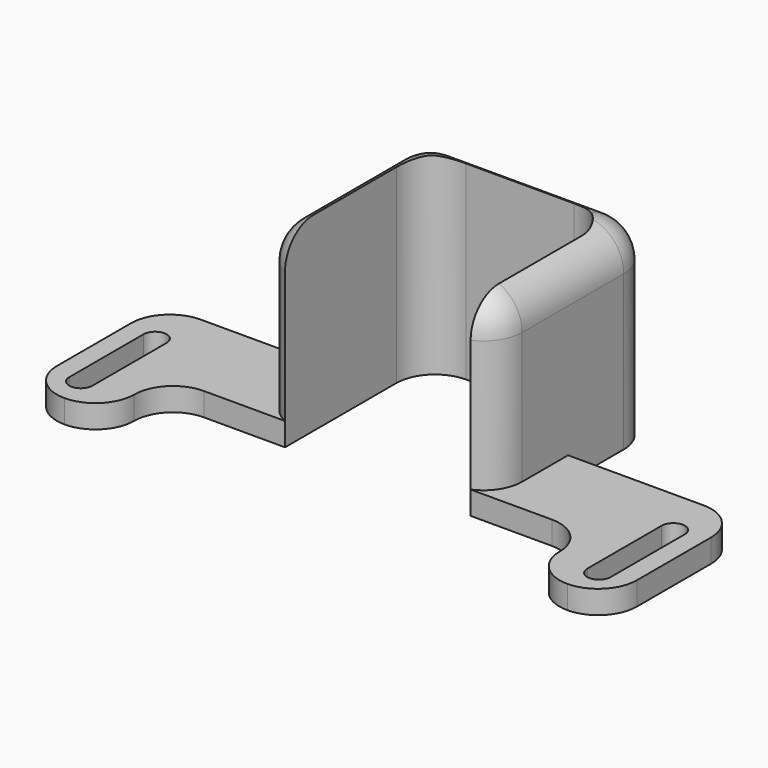
from build123d import *

# Parameters (mm, degrees)
F2_DEPTH     = 25
F3_DEPTH     = 3
F4_DEPTH     = 25
F5_R         = 4.99999
F6_T1_DEPTH  = 25
F6_T3_DEPTH  = 25
F6_T5_DEPTH  = 50
F6_T7_DEPTH  = 33.4564392374
F6_T9_DEPTH  = 50
F6_T11_DEPTH = 33.4564392374
F7_T1_DEPTH  = 16.417424305
F7_T3_DEPTH  = 20
F7_T6_ANGLE  = 89.9999999974
F7_T8_ANGLE  = 89.9999999974
F7_T10_ANGLE = 209.6926070845
F7_T12_ANGLE = 209.6926070845


# Not quite as in the source:
# - a fillet or chamfer that OpenCascade refuses, or shapes differently, is made with other operations: its cross-section is extruded or revolved along the edge and cut away or added
# - a fillet or chamfer is up to 0.001 mm smaller than in the source, because OpenCascade refuses the exact size


with BuildPart() as f2:
    # F0 (on Top) → F2 (new body)
    with BuildSketch(Plane.XY):
        Polygon((15, 36), (0, 36), (-15, 36), (-15, 22), (-15, 10), (-12, 10), (-12, 33), (0, 33), (12, 33), (12, 10), (15, 10), (15, 22), align=None)
    extrude(amount=F2_DEPTH)

    # F0 (on Top) → F3 (join)
    with BuildSketch(Plane.XY):
        Polygon((-15, 10), (-15, 22), (-37.5, 22), (-37.5, 0), (-27.5, 0), (-27.5, 10), align=None)
        Polygon((37.5, 22), (15, 22), (15, 10), (27.5, 10), (27.5, 0), (37.5, 0), align=None)
    extrude(amount=F3_DEPTH)

    # F1 (on Top) → F4 (cut)
    with BuildSketch(Plane.XY):
        with BuildLine():
            Line((35, 3.8767794613), (35, 15.8767794613))
            ThreePointArc((35, 15.8767794613), (33.5, 17.3767794613), (32, 15.8767794613))
            Line((32, 15.8767794613), (32, 3.8767794613))
            ThreePointArc((32, 3.8767794613), (33.5, 2.3767794613), (35, 3.8767794613))
        make_face()
        with BuildLine():
            ThreePointArc((-32, 15.8767794613), (-33.5, 17.3767794613), (-35, 15.8767794613))
            Line((-35, 15.8767794613), (-35, 3.8767794613))
            ThreePointArc((-35, 3.8767794613), (-33.5, 2.3767794613), (-32, 3.8767794613))
            Line((-32, 3.8767794613), (-32, 15.8767794613))
        make_face()
    extrude(amount=F4_DEPTH, mode=Mode.SUBTRACT)

    # F5 (radius 5 in the source; OpenCascade refuses exactly that, so slightly less here)
    f5_edges = [f2.edges().sort_by_distance(p)[0] for p in [
        (-37.5, 0, 1.5),
        (-27.5, 0, 1.5),
        (-37.5, 22, 1.5),
        (37.5, 22, 1.5),
        (37.5, 0, 1.5),
        (27.5, 0, 1.5),
        (27.5, 10, 1.5),
        (-27.5, 10, 1.5),
    ]]
    fillet(f5_edges, radius=F5_R)

    # F6: fillet of radius 5 on 6 edges, made by hand

    # F6_s2 → F6_t1 (join)
    with BuildSketch(Plane.XY):
        with BuildLine():
            ThreePointArc((12, 28), (10.5355339059, 31.5355339059), (7, 33))
            Line((7, 33), (12, 33))
            Line((12, 33), (12, 28))
        make_face()
    extrude(amount=F6_T1_DEPTH)

    # F6_s4 → F6_t3 (join)
    with BuildSketch(Plane.XY):
        with BuildLine():
            ThreePointArc((-7, 33), (-10.5355339059, 31.5355339059), (-12, 28))
            Line((-12, 28), (-12, 33))
            Line((-12, 33), (-7, 33))
        make_face()
    extrude(amount=F6_T3_DEPTH)

    # F6_s6 → F6_t5 (cut)
    with BuildSketch(Plane.XY.offset(-12.5)):
        with BuildLine():
            ThreePointArc((15, 31), (13.5355339059, 34.5355339059), (10, 36))
            Line((10, 36), (15, 36))
            Line((15, 36), (15, 31))
        make_face()
    extrude(amount=F6_T5_DEPTH, mode=Mode.SUBTRACT)

    # F6_s8 → F6_t7 (cut)
    with BuildSketch(Plane.XY.offset(3)):
        with BuildLine():
            ThreePointArc((12, 10), (14.1833001327, 11.8439629074), (15, 14.582575695))
            Line((15, 14.582575695), (15, 10))
            Line((15, 10), (12, 10))
        make_face()
    extrude(amount=F6_T7_DEPTH, mode=Mode.SUBTRACT)

    # F6_s10 → F6_t9 (cut)
    with BuildSketch(Plane.XY.offset(-12.5)):
        with BuildLine():
            ThreePointArc((-10, 36), (-13.5355339059, 34.5355339059), (-15, 31))
            Line((-15, 31), (-15, 36))
            Line((-15, 36), (-10, 36))
        make_face()
    extrude(amount=F6_T9_DEPTH, mode=Mode.SUBTRACT)

    # F6_s12 → F6_t11 (cut)
    with BuildSketch(Plane.XY.offset(3)):
        with BuildLine():
            ThreePointArc((-12, 10), (-14.1833001327, 11.8439629074), (-15, 14.582575695))
            Line((-15, 14.582575695), (-15, 10))
            Line((-15, 10), (-12, 10))
        make_face()
    extrude(amount=F6_T11_DEPTH, mode=Mode.SUBTRACT)

    # F7: fillet of radius 5 on 3 edges, made by hand

    # F7_s2 → F7_t1 (cut)
    with BuildSketch(Plane.XZ.offset(-31)):
        with BuildLine():
            ThreePointArc((-10, 25), (-13.5355339059, 23.5355339059), (-15, 20))
            Line((-15, 20), (-15, 25))
            Line((-15, 25), (-10, 25))
        make_face()
        with BuildLine():
            ThreePointArc((10, 25), (13.5355339059, 23.5355339059), (15, 20))
            Line((15, 20), (15, 25))
            Line((15, 25), (10, 25))
        make_face()
    extrude(amount=F7_T1_DEPTH, mode=Mode.SUBTRACT)

    # F7_s4 → F7_t3 (cut)
    with BuildSketch(Plane.YZ.offset(-10)):
        with BuildLine():
            ThreePointArc((31, 25), (34.5355339059, 23.5355339059), (36, 20))
            Line((36, 20), (36, 25))
            Line((36, 25), (31, 25))
        make_face()
    extrude(amount=F7_T3_DEPTH, mode=Mode.SUBTRACT)

    # F7_s5 → F7_t6 (revolve, cut)
    with BuildSketch(Plane.YZ.offset(9.9999999999)):
        with BuildLine():
            ThreePointArc((31, 25), (34.5355339059, 23.5355339059), (36, 20))
            Line((36, 20), (36, 25))
            Line((36, 25), (31, 25))
        make_face()
    revolve(axis=Axis((9.9999999999, 30.9999999999, 25), (0, 0, -1)), revolution_arc=F7_T6_ANGLE, mode=Mode.SUBTRACT)

    # F7_s7 → F7_t8 (revolve, cut)
    with BuildSketch(Plane.XZ.offset(-30.9999999999)):
        with BuildLine():
            ThreePointArc((-10, 25), (-13.5355339059, 23.5355339059), (-15, 20))
            Line((-15, 20), (-15, 25))
            Line((-15, 25), (-10, 25))
        make_face()
    revolve(axis=Axis((-9.9999999999, 30.9999999999, 25), (0, 0, -1)), revolution_arc=F7_T8_ANGLE, mode=Mode.SUBTRACT)

    # F7_s9 → F7_t10 (revolve, cut)
    with BuildSketch(Plane.XZ.offset(-14.5825756948)):
        with BuildLine():
            ThreePointArc((15, 20), (13.5355339059, 23.5355339059), (10, 25))
            Line((10, 25), (15, 25))
            Line((15, 25), (15, 20))
        make_face()
    revolve(axis=Axis((10.0000000002, 14.5825756948, 25), (0, 0, -1)), revolution_arc=F7_T10_ANGLE, mode=Mode.SUBTRACT)

    # F7_s11 → F7_t12 (revolve, cut)
    with BuildSketch(Plane(origin=(-8.7286422437, 15.307527957, 0), x_dir=(0, 0, 1), z_dir=(-0.4953465841, 0.8686954366, 0))):
        with BuildLine():
            ThreePointArc((25, -1.4635253083), (23.5355339059, 2.0720085977), (20, 3.5364746917))
            Line((20, 3.5364746917), (25, 3.5364746917))
            Line((25, 3.5364746917), (25, -1.4635253083))
        make_face()
    revolve(axis=Axis((-10.0000000002, 14.5825756948, 25), (0, 0, -1)), revolution_arc=F7_T12_ANGLE, mode=Mode.SUBTRACT)


solid = f2.part
